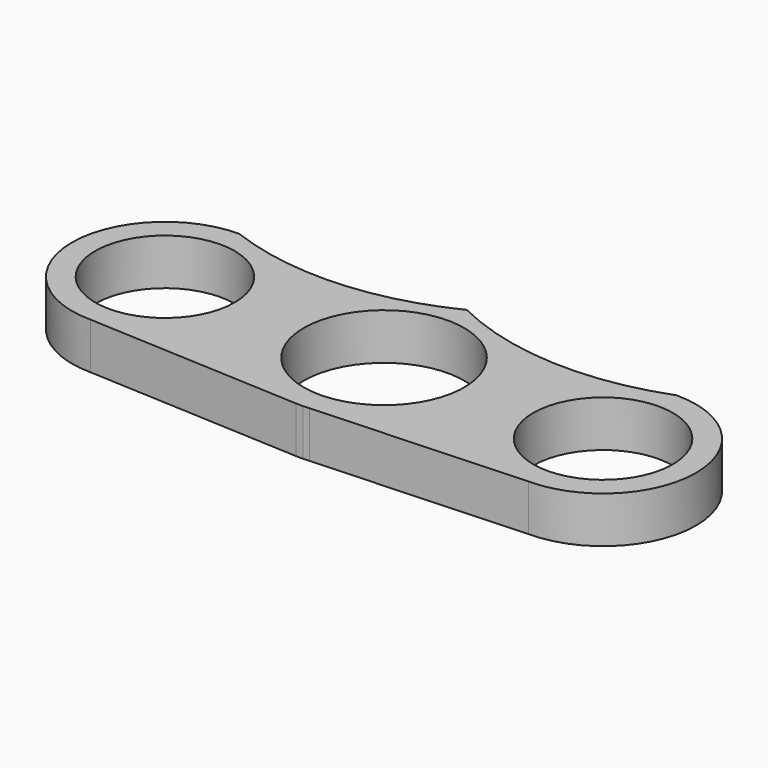
from build123d import *

# Parameters (mm, degrees)
F0_R     = 9.55
F1_DEPTH = 6.35
F3_DEPTH = 25


# Not quite as in the source:
# - a feature names something its author has since deleted; it is built from what else it names


with BuildPart() as f1:
    # F0 (on Top) → F1 (new body)
    with BuildSketch(Plane.XY):
        with BuildLine():
            Line((14.175, 0), (11, 0))
            ThreePointArc((11, 0), (0, -11), (-11, 0))
            Line((-11, 0), (-14.175, 0))
            ThreePointArc((-14.175, 0), (-10.265086005, -9.7754096748), (-0.6923002736, -14.1580840982))
            ThreePointArc((-0.6923002736, -14.1580840982), (-0.2241695179, -14.1732273328), (0.2442059858, -14.1728962614))
            Line((0.2442059858, -14.1728962614), (1.1329762166, -14.1296493195))
            ThreePointArc((1.1329762166, -14.1296493195), (10.4161068272, -9.6143301152), (14.175, 0))
        make_face()
        with BuildLine():
            ThreePointArc((-11, 0), (0, 11), (11, 0))
            Line((11, 0), (14.175, 0))
            ThreePointArc((14.175, 0), (10.4954430476, 9.5276597459), (1.3670564043, 14.1089256071))
            Line((1.3670564043, 14.1089256071), (0, 14.175))
            Line((0, 14.175), (-1.3670564043, 14.1089256071))
            ThreePointArc((-1.3670564043, 14.1089256071), (-10.4954430476, 9.5276597459), (-14.175, 0))
            Line((-14.175, 0), (-11, 0))
        make_face()
        with BuildLine():
            Line((17.275, 0), (14.175, 0))
            ThreePointArc((14.175, 0), (10.4161068272, -9.6143301152), (1.1329762166, -14.1296493195))
            Line((1.1329762166, -14.1296493195), (30, -12.725))
            ThreePointArc((30, -12.725), (21.0020662094, -8.9979337906), (17.275, 0))
        make_face()
        with BuildLine():
            ThreePointArc((1.3670564043, 14.1089256071), (10.4954430476, 9.5276597459), (14.175, 0))
            Line((14.175, 0), (17.275, 0))
            ThreePointArc((17.275, 0), (21.0020662094, 8.9979337906), (30, 12.725))
            Line((30, 12.725), (1.3670564043, 14.1089256071))
        make_face()
        with BuildLine():
            Line((-17.275, 0), (-14.175, 0))
            ThreePointArc((-14.175, 0), (-10.4954430476, 9.5276597459), (-1.3670564043, 14.1089256071))
            Line((-1.3670564043, 14.1089256071), (-30, 12.725))
            ThreePointArc((-30, 12.725), (-21.0020662094, 8.9979337906), (-17.275, 0))
        make_face()
        with BuildLine():
            ThreePointArc((-0.6923002736, -14.1580840982), (-10.265086005, -9.7754096748), (-14.175, 0))
            Line((-14.175, 0), (-17.275, 0))
            ThreePointArc((-17.275, 0), (-21.0020662094, -8.9979337906), (-30, -12.725))
            Line((-30, -12.725), (-0.6923002736, -14.1580840982))
        make_face()
        with BuildLine():
            ThreePointArc((30, 12.725), (21.0020662094, 8.9979337906), (17.275, 0))
            ThreePointArc((17.275, 0), (21.0020662094, -8.9979337906), (30, -12.725))
            ThreePointArc((30, -12.725), (38.9979337906, -8.9979337906), (42.725, 0))
            ThreePointArc((42.725, 0), (38.9979337906, 8.9979337906), (30, 12.725))
        make_face()
        with BuildLine():
            ThreePointArc((39.55, 0), (30, -9.55), (20.45, 0))
            ThreePointArc((20.45, 0), (30, 9.55), (39.55, 0))
        make_face(mode=Mode.SUBTRACT)
        with BuildLine():
            ThreePointArc((-30, -12.725), (-21.0020662094, -8.9979337906), (-17.275, 0))
            ThreePointArc((-17.275, 0), (-21.0020662094, 8.9979337906), (-30, 12.725))
            ThreePointArc((-30, 12.725), (-42.725, 0), (-30, -12.725))
        make_face()
        with Locations((-30, 0)):
            Circle(F0_R, mode=Mode.SUBTRACT)
    extrude(amount=F1_DEPTH)

    # F2 (on Top) → F3 (cut)
    with BuildSketch(Plane.XY):
        with BuildLine():
            ThreePointArc((-0.0002806461, 14.1748610267), (-20.9243917712, 47.820811609), (-0.0002806461, 81.4667621913))
            ThreePointArc((-0.0002806461, 81.4667621913), (-54.2064032082, 47.820811609), (-0.0002806461, 14.1748610267))
        make_face()
        with BuildLine():
            ThreePointArc((-0.0002806461, 14.1748610267), (15.2384059917, 28.0205677125), (20.8838914193, 47.820811609))
            ThreePointArc((20.8838914193, 47.820811609), (15.2384059917, 67.6210555055), (-0.0002806461, 81.4667621913))
            ThreePointArc((-0.0002806461, 81.4667621913), (-20.9243917712, 47.820811609), (-0.0002806461, 14.1748610267))
        make_face()
        with BuildLine():
            ThreePointArc((-0.0002806461, 81.4667621913), (15.2384059917, 67.6210555055), (20.8838914193, 47.820811609))
            ThreePointArc((20.8838914193, 47.820811609), (15.2384059917, 28.0205677125), (-0.0002806461, 14.1748610267))
            ThreePointArc((-0.0002806461, 14.1748610267), (36.3997744183, 15.9650923463), (54.1023755584, 47.820811609))
            ThreePointArc((54.1023755584, 47.820811609), (36.3997744183, 79.6765308717), (-0.0002806461, 81.4667621913))
        make_face()
    extrude(amount=F3_DEPTH, mode=Mode.SUBTRACT)


solid = f1.part
